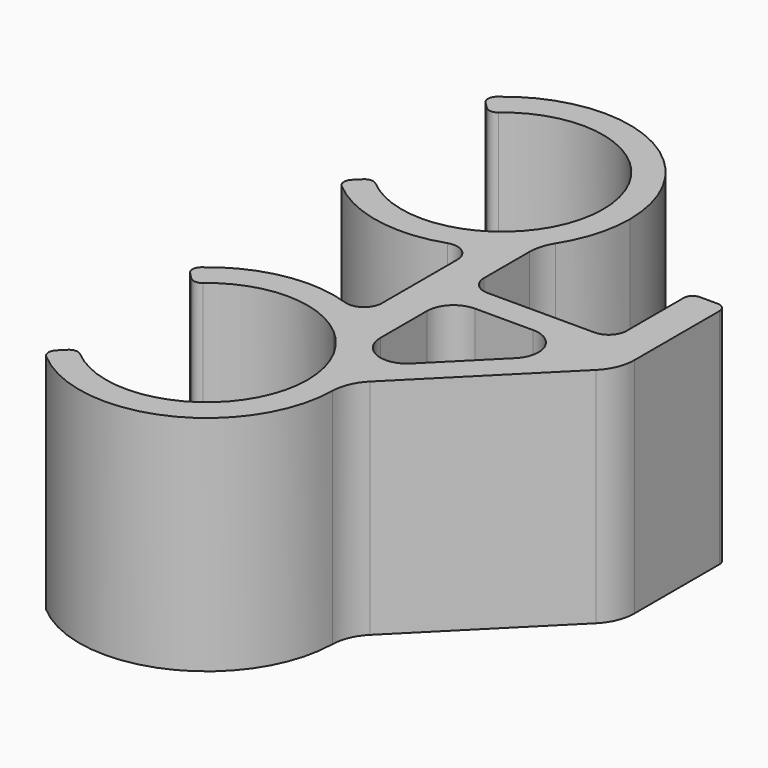
from build123d import *

# Parameters (mm, degrees)
F1_DEPTH    = 25
F2_T4_DEPTH = 25
F3_R        = 2
F4_R        = 1
F5_R        = 5
F6_R        = 2
F8_DEPTH    = 25.001
F9_R        = 3


# Not quite as in the source:
# - a fillet or chamfer that OpenCascade refuses, or shapes differently, is made with other operations: its cross-section is extruded or revolved along the edge and cut away or added


with BuildPart() as f1:
    # F0 (on Top) → F1 (new body)
    with BuildSketch(Plane.XY):
        with BuildLine():
            ThreePointArc((11.3, -11.9364390799), (9.4662629179, -9.9817974282), (7.3, -8.4036590808))
            Line((7.3, -8.4036590808), (7.3, -12.0744565389))
            ThreePointArc((7.3, -12.0744565389), (10.2513413756, -15.9460542704), (11.3, -20.7))
            Line((11.3, -20.7), (11.3, -11.9364390799))
        make_face()
        with BuildLine():
            ThreePointArc((11.3, 11.9364390799), (9.4662629179, 9.9817974282), (7.3, 8.4036590808))
            Line((7.3, 8.4036590808), (7.3, -8.4036590808))
            ThreePointArc((7.3, -8.4036590808), (9.4662629179, -9.9817974282), (11.3, -11.9364390799))
            Line((11.3, -11.9364390799), (11.3, -2))
            Line((11.3, -2), (11.3, 2))
            Line((11.3, 2), (11.3, 11.9364390799))
        make_face()
        with BuildLine():
            ThreePointArc((11.3, 20.7), (10.2513413756, 15.9460542704), (7.3, 12.0744565389))
            Line((7.3, 12.0744565389), (7.3, 8.4036590808))
            ThreePointArc((7.3, 8.4036590808), (9.4662629179, 9.9817974282), (11.3, 11.9364390799))
            Line((11.3, 11.9364390799), (11.3, 20.7))
        make_face()
        with BuildLine():
            ThreePointArc((-7.9903066274, 28.6903066274), (4.3243227857, 31.1398387174), (11.3, 20.7))
            Line((11.3, 20.7), (11.3, 11.9364390799))
            ThreePointArc((11.3, 11.9364390799), (13.5292276202, 16.0685855292), (14.3, 20.7))
            ThreePointArc((14.3, 20.7), (5.4723730828, 33.9114773149), (-10.111626971, 30.811626971))
            Line((-10.111626971, 30.811626971), (-7.9903066274, 28.6903066274))
        make_face()
        with BuildLine():
            Line((7.3, 8.4036590808), (7.3, 12.0744565389))
            ThreePointArc((7.3, 12.0744565389), (-0.4690546543, 9.4097392532), (-7.9903066274, 12.7096933726))
            Line((-7.9903066274, 12.7096933726), (-10.111626971, 10.588373029))
            ThreePointArc((-10.111626971, 10.588373029), (-1.7803244971, 6.5112564092), (7.3, 8.4036590808))
        make_face()
        with BuildLine():
            Line((7.3, -12.0744565389), (7.3, -8.4036590808))
            ThreePointArc((7.3, -8.4036590808), (-1.7803244971, -6.5112564092), (-10.111626971, -10.588373029))
            Line((-10.111626971, -10.588373029), (-7.9903066274, -12.7096933726))
            ThreePointArc((-7.9903066274, -12.7096933726), (-0.4690546543, -9.4097392532), (7.3, -12.0744565389))
        make_face()
        with BuildLine():
            ThreePointArc((14.3, -20.7), (13.5292276202, -16.0685855292), (11.3, -11.9364390799))
            Line((11.3, -11.9364390799), (11.3, -20.7))
            ThreePointArc((11.3, -20.7), (4.3243227857, -31.1398387174), (-7.9903066274, -28.6903066274))
            Line((-7.9903066274, -28.6903066274), (-10.111626971, -30.811626971))
            ThreePointArc((-10.111626971, -30.811626971), (5.4723730828, -33.9114773149), (14.3, -20.7))
        make_face()
        Polygon((27.3, 2), (11.3, 2), (11.3, -2), (31.3, -2), (31.3, 13), (27.3, 13), align=None)
    extrude(amount=F1_DEPTH)

    # F2: chamfer of 20 on 1 edges, made by hand


with BuildPart() as f2_tool2:
    # F2_s3 → F2_t4 (new body)
    with BuildSketch(Plane.XY):
        Polygon((11.3, -22), (31.3, -2), (11.3, -2), align=None)
    extrude(amount=F2_T4_DEPTH)

    split(bisect_by=Plane.YZ.offset(31.3), keep=Keep.BOTTOM)


with BuildPart() as f1_1:
    add(f1.part)

    # F2_t1: union F2_tool2
    add(f2_tool2.part)

    # F3
    f3_edges = [f1_1.edges().sort_by_distance(p)[0] for p in [
        (27.3, 2, 12.5),
        (11.3, 2, 12.5),
    ]]
    fillet(f3_edges, radius=F3_R)

    # F4
    f4_edges = [f1_1.edges().sort_by_distance(p)[0] for p in [
        (31.3, 13, 12.5),
        (27.3, 13, 12.5),
        (-7.990307, -12.709693, 12.5),
        (-10.111627, -10.588373, 12.5),
        (-7.990307, -28.690307, 12.5),
        (-10.111627, -30.811627, 12.5),
        (-10.111627, 10.588373, 12.5),
        (-7.990307, 12.709693, 12.5),
        (-7.990307, 28.690307, 12.5),
        (-10.111627, 30.811627, 12.5),
    ]]
    fillet(f4_edges, radius=F4_R)

    # F5
    f5_edges = [f1_1.edges().sort_by_distance(p)[0] for p in [
        (11.3, 11.936439, 12.5),
        (31.3, -2, 12.5),
        (14.209172, -19.090828, 12.5),
    ]]
    fillet(f5_edges, radius=F5_R)

    # F6
    f6_edges = [f1_1.edges().sort_by_distance(p)[0] for p in [
        (7.3, 8.403659, 12.5),
        (7.3, -8.403659, 12.5),
    ]]
    fillet(f6_edges, radius=F6_R)

    # F7 (on face) → F8 (cut, through all)
    with BuildSketch(Plane.XY.offset(25)):
        Polygon((28.0573593129, -1), (11.3, -1), (11.3, -17.7573593129), align=None)
    extrude(amount=-F8_DEPTH, mode=Mode.SUBTRACT)

    # F9
    f9_edges = [f1_1.edges().sort_by_distance(p)[0] for p in [
        (11.3, -1, 12.5),
        (28.057359, -1, 12.5),
        (11.3, -17.757359, 12.5),
    ]]
    fillet(f9_edges, radius=F9_R)


solid = f1_1.part
